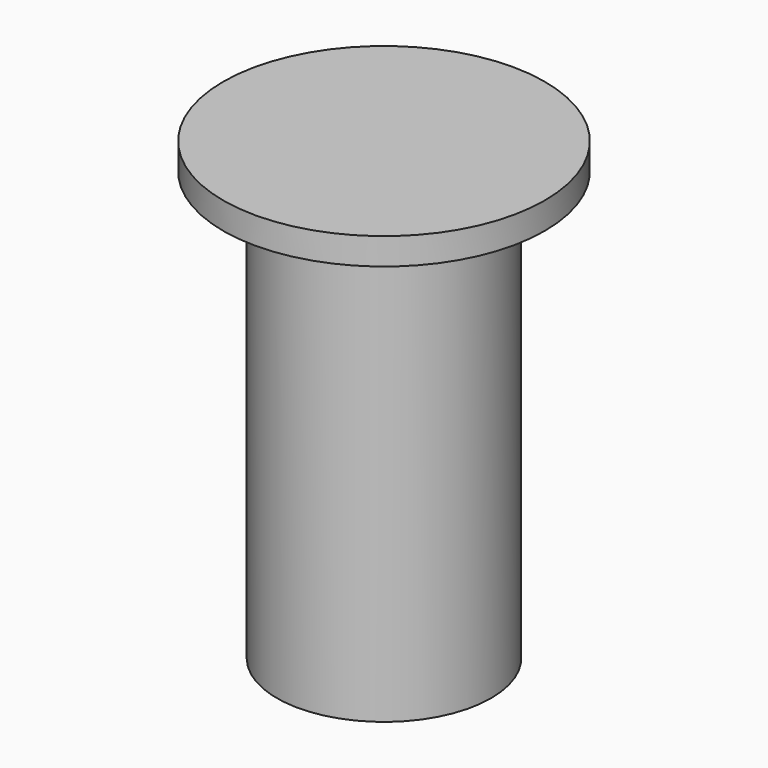
from build123d import *

# Parameters (mm, degrees)
F0_R     = 9.525
F1_DEPTH = 1.5875
F2_R     = 6.35
F3_DEPTH = 25.4


# Not quite as in the source:
# - a length typed as a fraction of an inch, garbled in the dataset ("3 / 203.2 mm" for 3/8 in), is restored


with BuildPart() as f1:
    # F0 (on Top) → F1 (new body)
    with BuildSketch(Plane.XY):
        Circle(F0_R)
    extrude(amount=F1_DEPTH)

    # F2 (on face) → F3 (join)
    with BuildSketch(Plane(origin=(0, 0, 0), x_dir=(1, 0, 0), z_dir=(0, 0, -1))):
        Circle(F2_R)
    extrude(amount=F3_DEPTH)


solid = f1.part
